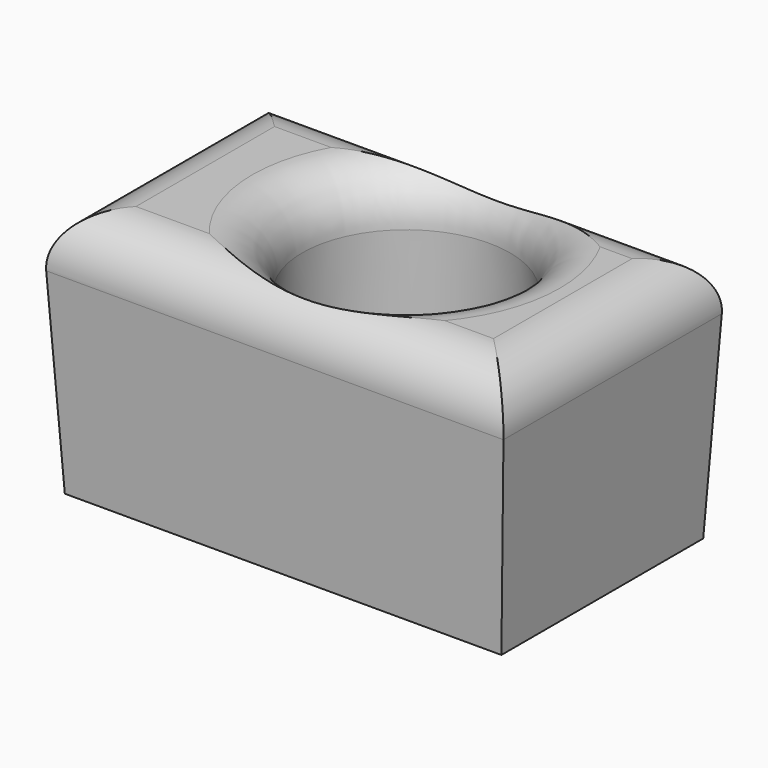
from build123d import *

# Parameters (mm, degrees)
F0_W        = 44.4304826669
F0_H        = 25.670937961
F1_DEPTH    = 25.4
F1_TAPER    = -3
F2_R        = 10.2925338698
F3_DEPTH    = 25.4
F3_TAPER    = -3
F4_T1_DEPTH = 73.8588130367
F4_T3_DEPTH = 55.0992683307


# Not quite as in the source:
# - a fillet or chamfer that OpenCascade refuses, or shapes differently, is made with other operations: its cross-section is extruded or revolved along the edge and cut away or added


with BuildPart() as f1:
    # F0 (on Top) → F1 (new body)
    with BuildSketch(Plane.XY):
        with Locations((-15.0602816138, -10.6690136017)):
            Rectangle(F0_W, F0_H)
    extrude(amount=F1_DEPTH, taper=F1_TAPER)

    # F2 (on face) → F3 (cut)
    with BuildSketch(Plane.XY.offset(25.4)):
        with Locations((-13.8062266633, -9.4221020117)):
            Circle(F2_R)
    extrude(amount=-F3_DEPTH, taper=F3_TAPER, mode=Mode.SUBTRACT)

    # F4: fillet of radius 5.08 on 5 edges, made by hand

    # F4_s2 → F4_t1 (cut)
    with BuildSketch(Plane.YZ.offset(-51.9896881322)):
        with BuildLine():
            ThreePointArc((-19.4824371396, 25.4), (-23.1673389443, 23.8168412445), (-24.5554751761, 20.0541333423))
            Line((-24.5554751761, 20.0541333423), (-24.835640176, 25.4))
            Line((-24.835640176, 25.4), (-19.4824371396, 25.4))
        make_face()
        with BuildLine():
            ThreePointArc((3.2174479727, 20.0541333423), (1.8293117409, 23.8168412445), (-1.8555900639, 25.4))
            Line((-1.8555900639, 25.4), (3.4976129725, 25.4))
            Line((3.4976129725, 25.4), (3.2174479727, 20.0541333423))
        make_face()
    extrude(amount=F4_T1_DEPTH, mode=Mode.SUBTRACT)

    # F4_s4 → F4_t3 (cut)
    with BuildSketch(Plane.XZ.offset(-16.8806205636)):
        with BuildLine():
            ThreePointArc((8.2059523135, 20.0541333423), (6.8178160817, 23.8168412445), (3.132914277, 25.4))
            Line((3.132914277, 25.4), (8.4861173134, 25.4))
            Line((8.4861173134, 25.4), (8.2059523135, 20.0541333423))
        make_face()
        with BuildLine():
            ThreePointArc((-33.2534775047, 25.4), (-36.9383793094, 23.8168412445), (-38.3265155412, 20.0541333423))
            Line((-38.3265155412, 20.0541333423), (-38.6066805411, 25.4))
            Line((-38.6066805411, 25.4), (-33.2534775047, 25.4))
        make_face()
    extrude(amount=F4_T3_DEPTH, mode=Mode.SUBTRACT)

    # F4_s5 → F4_t6 (revolve, cut)
    with BuildSketch(Plane.XZ.offset(9.4221020117)):
        with BuildLine():
            ThreePointArc((1.8395102429, 25.4), (-1.8453915618, 23.8168412445), (-3.2335277936, 20.0541333423))
            Line((-3.2335277936, 20.0541333423), (-3.5136927935, 25.4))
            Line((-3.5136927935, 25.4), (1.8395102429, 25.4))
        make_face()
    revolve(axis=Axis((-13.8062266633, -9.4221020117, 25.4), (0, 0, -1)), mode=Mode.SUBTRACT)


solid = f1.part
